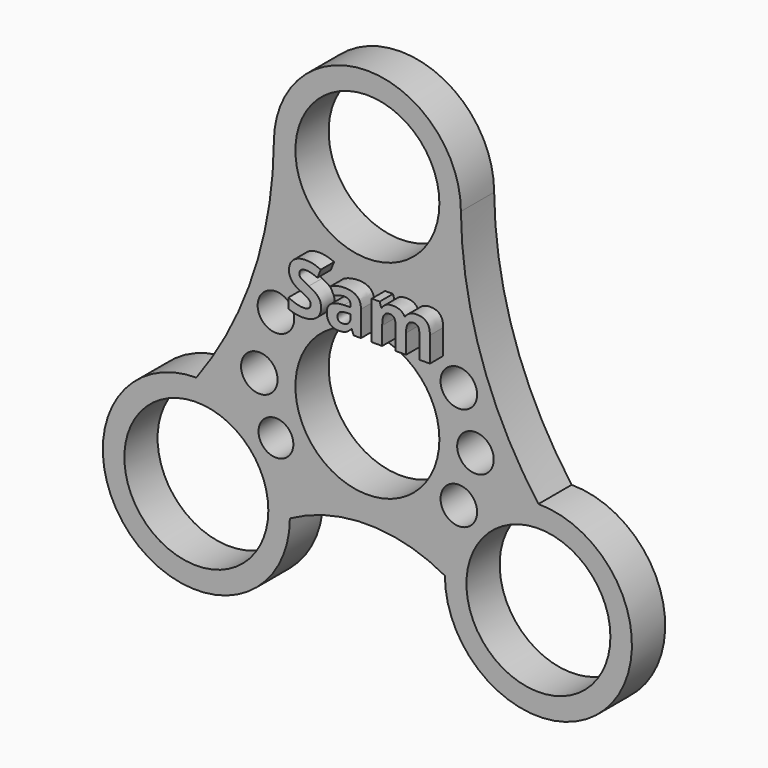
from build123d import *

# Parameters (mm, degrees)
F0_R         = 14.2875
F0_R_2       = 10.9982
F1_DEPTH     = 6.35
F2_TEXT_SIZE = 10.7207817778
F3_DEPTH     = 2.54
F4_R         = 2.794
F4_R_2       = 2.6614006185
F5_DEPTH     = 25.4


# Not quite as in the source:
# - Text() gives the source's letters only with a copy of the font that has no kerning and outlines rounded to 1/6400 em; it was checked with that copy


with BuildPart() as f1:
    # F0 (on Front) → F1 (new body)
    with BuildSketch(Plane.XZ):
        with BuildLine():
            ThreePointArc((26.1281930785, -3.7507933353), (17.4139339607, 13.0677407393), (14.2875, 31.75))
            ThreePointArc((14.2875, 31.75), (0, 17.4625), (-14.2875, 31.75))
            ThreePointArc((-14.2875, 31.75), (-17.4160613033, 13.0697568488), (-26.131156576, -3.7465))
            ThreePointArc((-26.131156576, -3.7465), (-16.0283684398, -7.9312118638), (-11.843656576, -18.034))
            ThreePointArc((-11.843656576, -18.034), (-0.0009258922, -14.9697424642), (11.8406930785, -18.0382933353))
            ThreePointArc((11.8406930785, -18.0382933353), (16.0254049423, -7.9355051991), (26.1281930785, -3.7507933353))
        make_face()
        Circle(F0_R, mode=Mode.SUBTRACT)
        with BuildLine():
            ThreePointArc((-14.2875, 31.75), (0, 17.4625), (14.2875, 31.75))
            ThreePointArc((14.2875, 31.75), (0, 46.0375), (-14.2875, 31.75))
        make_face()
        with Locations((0, 31.75)):
            Circle(F0_R_2, mode=Mode.SUBTRACT)
        with BuildLine():
            ThreePointArc((40.4156930785, -18.0382933353), (36.2309812147, -7.9355051991), (26.1281930785, -3.7507933353))
            ThreePointArc((26.1281930785, -3.7507933353), (16.0254049423, -7.9355051991), (11.8406930785, -18.0382933353))
            ThreePointArc((11.8406930785, -18.0382933353), (26.1281930785, -32.3257933353), (40.4156930785, -18.0382933353))
        make_face()
        with Locations((26.1281930785, -18.0382933353)):
            Circle(F0_R_2, mode=Mode.SUBTRACT)
        Circle(F0_R)
        Circle(F0_R_2, mode=Mode.SUBTRACT)
        with BuildLine():
            ThreePointArc((-11.843656576, -18.034), (-16.0283684398, -7.9312118638), (-26.131156576, -3.7465))
            ThreePointArc((-26.131156576, -3.7465), (-36.2339447122, -28.1367881362), (-11.843656576, -18.034))
        make_face()
        with Locations((-26.131156576, -18.034)):
            Circle(F0_R_2, mode=Mode.SUBTRACT)
    extrude(amount=F1_DEPTH)

    # F2 (on face) → F3 (join)
    with BuildSketch(Plane.XZ.offset(6.35)):
        with Locations((-10.522912954, 11.43)):
            Text('Sam', F2_TEXT_SIZE, font='Open Sans', font_style=FontStyle.BOLD, text_align=(TextAlign.LEFT, TextAlign.BOTTOM))
    extrude(amount=F3_DEPTH)

    # F4 (on face) → F5 (cut)
    with BuildSketch(Plane.XZ.offset(6.35)):
        with Locations((-13.97, 9.013770081)):
            Circle(F4_R)
        with Locations((-16.51, 0)):
            Circle(F4_R)
        with Locations((-13.97, -7.8975260258)):
            Circle(F4_R_2)
        with Locations((13.97, -7.8975260258)):
            Circle(F4_R)
        with Locations((16.51, 0)):
            Circle(F4_R)
        with Locations((13.97, 7.9178729108)):
            Circle(F4_R)
    extrude(amount=-F5_DEPTH, mode=Mode.SUBTRACT)


solid = f1.part
